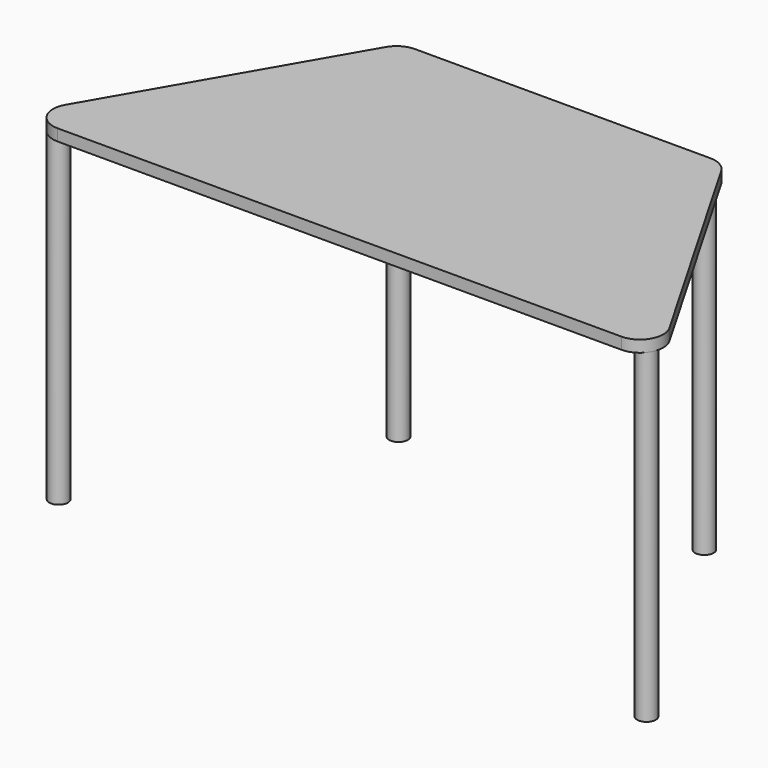
from build123d import *

# Parameters (mm, degrees)
F2_DEPTH = 25
F1_R     = 20
F3_DEPTH = 700
F4_R     = 49.99999


# Not quite as in the source:
# - a fillet or chamfer is up to 0.001 mm smaller than in the source, because OpenCascade refuses the exact size


with BuildPart() as f2:
    # F0 (on Top) → F2 (new body)
    with BuildSketch(Plane.XY):
        Polygon((0, 0), (0, 300), (-346.4101615138, 300), (-692.8203230276, -300), (0, -300), align=None)
        Polygon((346.4101615138, 300), (0, 300), (0, 0), (0, -300), (692.8203230276, -300), align=None)
    extrude(amount=F2_DEPTH)

    # F1 (on Top) → F3 (join)
    with BuildSketch(Plane.XY):
        with Locations((-328.9101615138, 269.6891108675)):
            Circle(F1_R)
        with Locations((-632.1985447626, -265)):
            Circle(F1_R)
        with Locations((328.9101615138, 269.6891108675)):
            Circle(F1_R)
        with Locations((632.1985447626, -265)):
            Circle(F1_R)
    extrude(amount=-F3_DEPTH)

    # F4 (radius 50 in the source; OpenCascade refuses exactly that, so slightly less here)
    f4_edges = [f2.edges().sort_by_distance(p)[0] for p in [
        (-692.820323, -300, 12.5),
        (-346.410162, 300, 12.5),
        (346.410162, 300, 12.5),
        (692.820323, -300, 12.5),
    ]]
    fillet(f4_edges, radius=F4_R)


solid = f2.part
